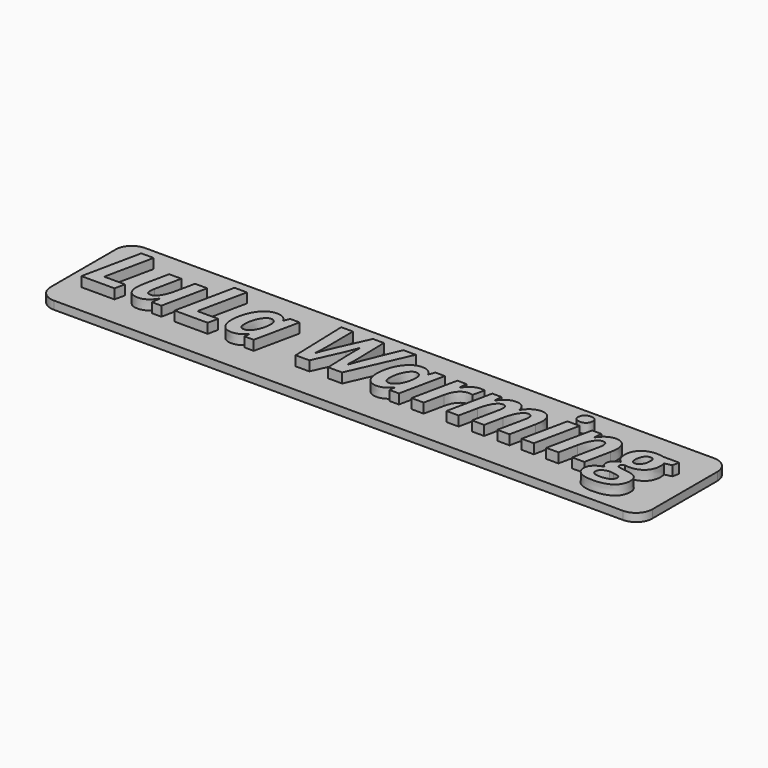
from build123d import *

# Parameters (mm, degrees)
F1_DEPTH     = 0.5
F2_TEXT_SIZE = 5.1070427031
F3_DEPTH     = 0.6


# Not quite as in the source:
# - Text() gives the source's letters only with a copy of the font that has no kerning and outlines rounded to 1/6400 em; it was checked with that copy


with BuildPart() as f1:
    # F0 (on Top) → F1 (new body)
    with BuildSketch(Plane.XY):
        with BuildLine():
            Line((17.5, 3.5), (-17.5, 3.5))
            ThreePointArc((-17.5, 3.5), (-18.2071067812, 3.2071067812), (-18.5, 2.5))
            Line((-18.5, 2.5), (-18.5, -2.5))
            ThreePointArc((-18.5, -2.5), (-18.2071067812, -3.2071067812), (-17.5, -3.5))
            Line((-17.5, -3.5), (17.5, -3.5))
            ThreePointArc((17.5, -3.5), (18.2071067812, -3.2071067812), (18.5, -2.5))
            Line((18.5, -2.5), (18.5, 2.5))
            ThreePointArc((18.5, 2.5), (18.2071067812, 3.2071067812), (17.5, 3.5))
        make_face()
    extrude(amount=F1_DEPTH)

    # F2 (on face) → F3 (join)
    with BuildSketch(Plane.XY.offset(0.5)):
        with Locations((-17.4697993834, -1.5921797906)):
            Text('LuLa Warming', F2_TEXT_SIZE, font='Open Sans', font_style=FontStyle.BOLDITALIC, text_align=(TextAlign.LEFT, TextAlign.BOTTOM))
    extrude(amount=F3_DEPTH)


solid = f1.part
